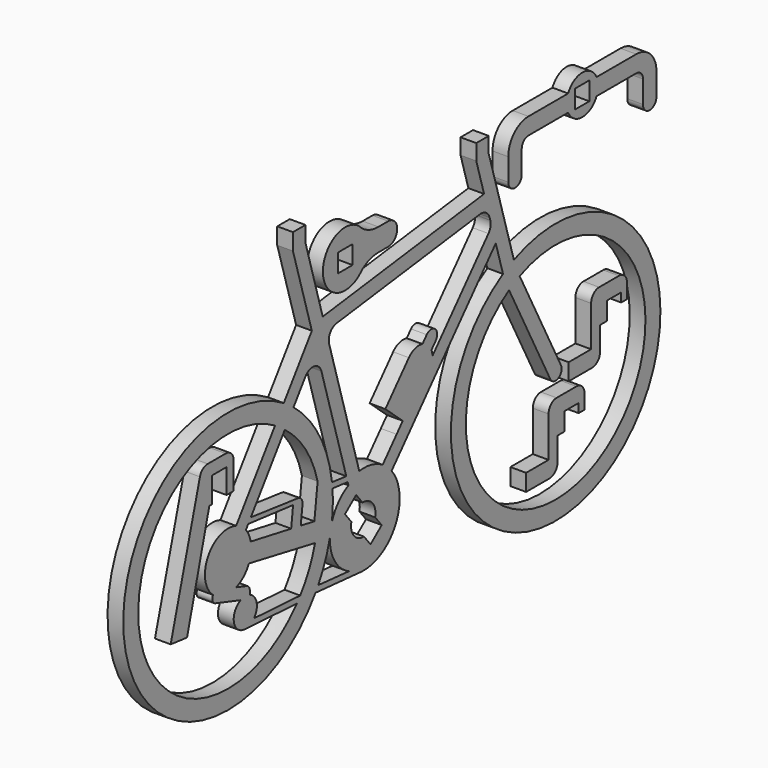
from build123d import *

# Parameters (mm, degrees)
F2_DEPTH = 2.8
F1_W     = 3.286
F1_H     = 3.286
F1_W_2   = 3.2
F1_H_2   = 3.2858568893


# Not quite as in the source:
# - ends of sketch curves that miss each other by under 0.0002 mm in the source are joined
# - a feature names something its author has since deleted; it is built from what else it names


with BuildPart() as f2:
    # F1 (on Right) → F2 (new body)
    with BuildSketch(Plane.YZ):
        with BuildLine():
            Line((-32.7810810621, 40.0630099882), (-28.5785464468, 25.854345194))
            Line((-28.5785464468, 25.854345194), (-34.8295213879, 17.0517607704))
            ThreePointArc((-34.8295213879, 17.0517607704), (-70.0441528649, -7.6634310767), (-27.7561804721, -15.577871613))
            Line((-27.7561804721, -15.577871613), (-17.4309209468, -16.4342678025))
            ThreePointArc((-17.4309209468, -16.4342678025), (-17.421352009, -16.4349690955), (-17.4117713764, -16.4354866475))
            ThreePointArc((-17.4117713764, -16.4354866475), (-9.8783278177, -12.024945839), (-10.8100300989, -3.3452239002))
            Line((-10.8100300989, -3.3452239002), (12.3781786089, 22.9225390659))
            Line((12.3781786089, 22.9225390659), (13.9960358427, 17.4527707038))
            ThreePointArc((13.9960358427, 17.4527707038), (36.2440392418, -23.5369879191), (16.4146126558, 18.6758988393))
            Line((16.4146126558, 18.6758988393), (14.2536723845, 25.9817614853))
            ThreePointArc((14.2536723845, 25.9817614853), (14.2515405676, 25.989045047), (14.2493673209, 25.9963163545))
            Line((14.2493673209, 25.9963163545), (12.7777300944, 30.9717335764))
            Line((12.7777300944, 30.9717335764), (10.8173713638, 37.5995357396))
            Line((10.8173713638, 37.5995357396), (10.8173713638, 40.3995357399))
            Line((10.8173713638, 40.3995357399), (8.037018366, 40.3995357399))
            Line((8.037018366, 40.3995357399), (8.037018366, 37.5995357399))
            Line((8.037018366, 37.5995357399), (9.7773678827, 31.7155655707))
            Line((9.7773678827, 31.7155655707), (-26.1566620581, 27.0789083905))
            Line((-26.1566620581, 27.0789083905), (-30.0007321323, 40.2276701755))
            Line((-30.0007321323, 40.2276701755), (-30.0007321323, 43.0276701755))
            Line((-30.0007321323, 43.0276701755), (-32.7810810175, 43.0276701755))
            Line((-32.7810810175, 43.0276701755), (-32.7810810621, 40.0630099882))
        make_face()
        with BuildLine():
            ThreePointArc((-27.1589419206, -14.6239739066), (-25.6381564049, -11.5709515578), (-24.5785787783, -8.3288797973))
            ThreePointArc((-24.5785787783, -8.3288797973), (-23.4485868958, -12.4014570535), (-20.3032664054, -15.2245273988))
            Line((-20.3032664054, -15.2245273988), (-27.1589419206, -14.6239739066))
        make_face(mode=Mode.SUBTRACT)
        with BuildLine():
            Line((-36.7690909191, 14.3204708989), (-45.438959238, 2.1116157144))
            ThreePointArc((-45.438959238, 2.1116157144), (-51.679021575, -0.1114645339), (-50.5741858599, -6.6429116785))
            ThreePointArc((-50.5741858599, -6.6429116785), (-50.7001368643, -7.5358957288), (-50.0559554, -8.1670172786))
            Line((-50.0559554, -8.1670172786), (-44.4357401431, -9.9504751803))
            ThreePointArc((-44.4357401431, -9.9504751803), (-45.9475994843, -12.7053301629), (-43.682084094, -14.8830318549))
            Line((-43.682084094, -14.8830318549), (-43.4085644782, -14.8992046485))
            Line((-43.4085644782, -14.8992046485), (-31.9213599112, -15.5784253597))
            ThreePointArc((-31.9213599112, -15.5784253597), (-66.9726575865, -5.9191061127), (-36.7690909191, 14.3204708989))
        make_face(mode=Mode.SUBTRACT)
        with BuildLine():
            ThreePointArc((-45.417431414, -7.5410613439), (-43.7533998551, -6.5186996051), (-42.5893207169, -4.9505336974))
            Line((-42.5893207169, -4.9505336974), (-27.8742179451, -7.7233503042))
            ThreePointArc((-27.8742179451, -7.7233503042), (-29.1875288387, -11.3310895929), (-31.1661285889, -14.6213344633))
            Line((-31.1661285889, -14.6213344633), (-41.4453615912, -14.013539249))
            ThreePointArc((-41.4453615912, -14.013539249), (-40.8757428579, -11.7304415251), (-42.3931878811, -9.9320085072))
            Line((-42.3931878811, -9.9320085072), (-42.3931878811, -9.2324187691))
            ThreePointArc((-42.3931878811, -9.2324187691), (-42.5861622295, -8.6419628585), (-43.0905932927, -8.2794348124))
            Line((-43.0905932927, -8.2794348124), (-45.417431414, -7.5410613439))
        make_face(mode=Mode.SUBTRACT)
        with BuildLine():
            Line((-15.5088098858, -12.9576973057), (-16.9709924298, -11.149063212))
            ThreePointArc((-16.9709924298, -11.149063212), (-19.2224479888, -10.1072740955), (-19.7694541503, -7.6875301098))
            Line((-19.7694541503, -7.6875301098), (-21.2014292566, -5.9162608458))
            Line((-21.2014292566, -5.9162608458), (-18.7129342238, -3.9044476159))
            Line((-18.7129342238, -3.9044476159), (-17.2809591175, -5.67571688))
            ThreePointArc((-17.2809591175, -5.67571688), (-15.0295035586, -6.7175059964), (-14.4824973971, -9.1372499821))
            Line((-14.4824973971, -9.1372499821), (-13.0203148531, -10.9458840758))
            Line((-13.0203148531, -10.9458840758), (-15.5088098858, -12.9576973057))
        make_face(mode=Mode.SUBTRACT)
        with BuildLine():
            ThreePointArc((-20.4284332347, -1.7008787129), (-22.713034199, -3.5049348102), (-24.1327228009, -6.0462935497))
            ThreePointArc((-24.1327228009, -6.0462935497), (-23.9042746908, -3.4009611929), (-23.9777551737, -0.7467998497))
            Line((-23.9777551737, -0.7467998497), (-20.6010095051, -1.1174049345))
            Line((-20.6010095051, -1.1174049345), (-20.4284332347, -1.7008787129))
        make_face(mode=Mode.SUBTRACT)
        with BuildLine():
            ThreePointArc((-42.1876674295, -1.6755199445), (-42.5889328041, -0.4877747618), (-43.2651398515, 0.5679224243))
            Line((-43.2651398515, 0.5679224243), (-42.7367221094, 1.3120370351))
            Line((-42.7367221094, 1.3120370351), (-32.7536984043, 0.2163787562))
            Line((-32.7536984043, 0.2163787562), (-33.1812144267, -3.3188663768))
            Line((-33.1812144267, -3.3188663768), (-42.1876674295, -1.6755199445))
        make_face(mode=Mode.SUBTRACT)
        with BuildLine():
            Line((-31.6963693255, 0.8509632025), (-42.1651316758, 2.1169471643))
            Line((-42.1651316758, 2.1169471643), (-34.5952715328, 12.7767776084))
            ThreePointArc((-34.5952715328, 12.7767776084), (-29.9994401309, 7.8666759835), (-27.2914488726, 1.7105775773))
            Line((-27.2914488726, 1.7105775773), (-28.0136806178, -4.2617512446))
            Line((-28.0136806178, -4.2617512446), (-31.0443248868, -3.708770127))
            Line((-31.0443248868, -3.708770127), (-30.6536988323, -0.4785780739))
            ThreePointArc((-30.6536988323, -0.4785780739), (-30.8996770647, 0.402136694), (-31.6963693255, 0.8509632025))
        make_face(mode=Mode.SUBTRACT)
        with BuildLine():
            ThreePointArc((24.5326127574, -3.3329199604), (26.3299626073, -3.9019308276), (26.8989734744, -2.1045809777))
            Line((26.8989734744, -2.1045809777), (17.7069262182, 15.603641135))
            ThreePointArc((17.7069262182, 15.603641135), (34.9283354862, -20.4664558462), (15.3405655012, 14.3753021523))
            Line((15.3405655012, 14.3753021523), (24.5326127574, -3.3329199604))
        make_face(mode=Mode.SUBTRACT)
        with BuildLine():
            ThreePointArc((-29.9983734724, 19.2501011531), (-28.0396469956, 20.0648164886), (-26.4504948685, 18.6594816511))
            Line((-26.4504948685, 18.6594816511), (-20.9085424497, -0.0776477954))
            Line((-20.9085424497, -0.0776477954), (-24.0866021245, 0.2711510752))
            ThreePointArc((-24.0866021245, 0.2711510752), (-26.8907561473, 8.722170153), (-32.6557020014, 15.5080674802))
            Line((-32.6557020014, 15.5080674802), (-29.9983734724, 19.2501011531))
        make_face(mode=Mode.SUBTRACT)
        with BuildLine():
            Line((-18.0250834345, -0.4262562289), (-24.7288519992, 22.2389292241))
            ThreePointArc((-24.7288519992, 22.2389292241), (-24.4867438443, 23.8976541842), (-23.0672336955, 24.7892683327))
            Line((-23.0672336955, 24.7892683327), (8.8532049047, 28.9080418475))
            ThreePointArc((8.8532049047, 28.9080418475), (10.2006691115, 28.6002630517), (11.0266106326, 27.4920175106))
            Line((11.0266106326, 27.4920175106), (11.1717955661, 27.0011658215))
            ThreePointArc((11.1717955661, 27.0011658215), (11.2066686934, 26.0018903312), (10.7533788193, 25.1106575162))
            Line((10.7533788193, 25.1106575162), (-1.7245508843, 10.9755725718))
            ThreePointArc((-1.7245508843, 10.9755725718), (-1.7897327542, 11.4952481661), (-1.9443174541, 11.9956629641))
            Line((-1.9443174541, 11.9956629641), (-0.9945827645, 13.0715289795))
            ThreePointArc((-0.9945827646, 13.0715289795), (-1.1117489129, 14.9531537943), (-2.9933737277, 14.8359876459))
            Line((-2.9933737277, 14.8359876459), (-3.9431084172, 13.7601216304))
            ThreePointArc((-3.9431084172, 13.7601216304), (-5.5866841115, 13.7356227774), (-6.9705428385, 12.8485623057))
            Line((-6.9705428385, 12.8485623057), (-12.2077076552, 6.9158658319))
            Line((-12.2077076552, 6.9158658319), (-8.3300521573, 3.4928151103))
            Line((-8.3300521573, 3.4928151103), (-9.6983886135, 1.9427541226))
            Line((-9.6983886135, 1.9427541226), (-12.8088210603, -1.5807652347))
            ThreePointArc((-12.8088210603, -1.5807652347), (-15.3182270596, -0.5574540272), (-18.0250834345, -0.4262562289))
        make_face(mode=Mode.SUBTRACT)
    extrude(amount=F2_DEPTH)


with BuildPart() as f2b:
    # F1 (on Right) → F2, piece 2 (new body)
    with BuildSketch(Plane.YZ):
        with BuildLine():
            Line((26.1350085661, -17.0272199881), (26.1350085661, -12.8250569627))
            Line((26.1350085661, -12.8250569627), (27.6350085661, -12.8250569627))
            Line((27.6350085661, -12.8250569627), (27.6350085661, -9.6250569627))
            Line((27.6350085661, -9.6250569627), (30.8350085661, -9.6250569627))
            Line((30.8350085661, -9.6250569627), (30.8350085661, -11.2250569627))
            Line((30.8350085661, -11.2250569627), (32.1350085661, -11.2250569627))
            Line((32.1350085661, -11.2250569627), (32.1350085661, -8.6228939372))
            ThreePointArc((32.1350085661, -8.6228939372), (31.6084343077, -7.351631221), (30.3371715916, -6.8250569627))
            Line((30.3371715916, -6.8250569627), (26.1350085661, -6.8250569627))
            Line((26.1350085661, -6.8250569627), (25.9328455406, -6.8250569627))
            ThreePointArc((25.9328455406, -6.8250569627), (24.6615828245, -7.351631221), (24.1350085661, -8.6228939372))
            Line((24.1350085661, -8.6228939372), (24.1350085661, -15.8250569627))
            Line((24.1350085661, -15.8250569627), (19.1350085661, -15.8250569627))
            Line((19.1350085661, -15.8250569627), (19.1350085661, -18.8250569627))
            Line((19.1350085661, -18.8250569627), (24.3371715916, -18.8250569627))
            ThreePointArc((24.3371715916, -18.8250569627), (25.6084343077, -18.2984827043), (26.1350085661, -17.0272199881))
        make_face()
    extrude(amount=F2_DEPTH)


with BuildPart() as f2c:
    # F1 (on Right) → F2, piece 3 (new body)
    with BuildSketch(Plane.YZ):
        with BuildLine():
            Line((-47.7713023129, 14.3973374015), (-51.7613397022, 14.3973374015))
            ThreePointArc((-51.7613397022, 14.3973374015), (-52.8518038089, 14.0305013357), (-53.496568146, 13.077632186))
            Line((-53.496568146, 13.077632186), (-60.0158057756, -10.5528221893))
            Line((-60.0158057756, -10.5528221893), (-56.367214369, -10.9714387513))
            Line((-56.367214369, -10.9714387513), (-51.4058386912, 7.6636058447))
            Line((-51.4058386912, 7.6636058447), (-50.7571436434, 7.6636058447))
            Line((-50.7571436434, 7.6636058447), (-50.7571436434, 12.2000958209))
            Line((-50.7571436434, 12.2000958209), (-47.5571436434, 12.2000958209))
            Line((-47.5571436434, 12.2000958209), (-47.5571436434, 7.799523944))
            Line((-47.5571436434, 7.799523944), (-45.9734653383, 7.799523944))
            Line((-45.9734653383, 7.799523944), (-45.9734653383, 12.599500427))
            ThreePointArc((-45.9734653383, 12.599500427), (-46.5000395967, 13.8707631432), (-47.7713023129, 14.3973374015))
        make_face()
    extrude(amount=F2_DEPTH)


with BuildPart() as f2d:
    # F1 (on Right) → F2, piece 4 (new body)
    with BuildSketch(Plane.YZ):
        with BuildLine():
            ThreePointArc((-11.5660707645, 32.1164598398), (-9.5660707645, 34.1164598398), (-11.5660707645, 36.1164598398))
            Line((-11.5660707645, 36.1164598398), (-13.7510611544, 36.1164598398))
            ThreePointArc((-13.7510611544, 36.1164598398), (-15.6803701734, 36.4351072976), (-17.4047560543, 37.35720427))
            ThreePointArc((-17.4047560543, 37.35720427), (-26.1140103212, 34.1164598398), (-17.4047560543, 30.8757154096))
            ThreePointArc((-17.4047560543, 30.8757154096), (-15.6803701734, 31.7978123821), (-13.7510611544, 32.1164598398))
            Line((-13.7510611544, 32.1164598398), (-11.5660707645, 32.1164598398))
        make_face()
        with Locations((-21.1564369343, 34.1164598398)):
            Rectangle(F1_W, F1_H, mode=Mode.SUBTRACT)
    extrude(amount=F2_DEPTH)


with BuildPart() as f2e:
    # F1 (on Right) → F2, piece 5 (new body)
    with BuildSketch(Plane.YZ):
        with BuildLine():
            ThreePointArc((15.1628487238, 31.3657282359), (16.6628487238, 29.8657282359), (18.1628487238, 31.3657282359))
            Line((18.1628487238, 31.3657282359), (18.1628487238, 35.3657282359))
            ThreePointArc((18.1628487238, 35.3657282359), (18.602188552, 36.4263884077), (19.6628487238, 36.8657282359))
            Line((19.6628487238, 36.8657282359), (28.5005710636, 36.8657282359))
            ThreePointArc((28.5005710636, 36.8657282359), (31.6628487238, 34.8657282359), (34.825126384, 36.8657282359))
            Line((34.825126384, 36.8657282359), (43.6628487238, 36.8657282359))
            ThreePointArc((43.6628487238, 36.8657282359), (44.7235088956, 36.4263884077), (45.1628487238, 35.3657282359))
            Line((45.1628487238, 35.3657282359), (45.1628487238, 31.3657282359))
            ThreePointArc((45.1628487238, 31.3657282359), (46.6628487238, 29.8657282359), (48.1628487238, 31.3657282359))
            Line((48.1628487238, 31.3657282359), (48.1628487238, 35.3657282359))
            ThreePointArc((48.1628487238, 35.3657282359), (46.8448292391, 38.5477087513), (43.6628487238, 39.8657282359))
            Line((43.6628487238, 39.8657282359), (34.825126384, 39.8657282359))
            ThreePointArc((34.825126384, 39.8657282359), (31.6628487238, 41.8657282359), (28.5005710636, 39.8657282359))
            Line((28.5005710636, 39.8657282359), (19.6628487238, 39.8657282359))
            ThreePointArc((19.6628487238, 39.8657282359), (16.4808682084, 38.5477087513), (15.1628487238, 35.3657282359))
            Line((15.1628487238, 35.3657282359), (15.1628487238, 31.3657282359))
        make_face()
        with Locations((31.6199202791, 38.3657282359)):
            Rectangle(F1_W_2, F1_H_2, mode=Mode.SUBTRACT)
    extrude(amount=F2_DEPTH)


with BuildPart() as f2f:
    # F1 (on Right) → F2, piece 6 (new body)
    with BuildSketch(Plane.YZ):
        with BuildLine():
            Line((39.8146519543, 6.6714825634), (35.6124889288, 6.6714825634))
            Line((35.6124889288, 6.6714825634), (35.4103259033, 6.6714825634))
            ThreePointArc((35.4103259033, 6.6714825634), (34.1390631872, 6.144908305), (33.6124889288, 4.8736455889))
            Line((33.6124889288, 4.8736455889), (33.6124889288, -2.3285174366))
            Line((33.6124889288, -2.3285174366), (28.6124889288, -2.3285174366))
            Line((28.6124889288, -2.3285174366), (28.6124889288, -5.3285174366))
            Line((28.6124889288, -5.3285174366), (33.8146519543, -5.3285174366))
            ThreePointArc((33.8146519543, -5.3285174366), (35.0859146704, -4.8019431782), (35.6124889288, -3.5306804621))
            Line((35.6124889288, -3.5306804621), (35.6124889288, 0.6714825634))
            Line((35.6124889288, 0.6714825634), (37.1124889288, 0.6714825634))
            Line((37.1124889288, 0.6714825634), (37.1124889288, 3.8714825634))
            Line((37.1124889288, 3.8714825634), (40.3124889288, 3.8714825634))
            Line((40.3124889288, 3.8714825634), (40.3124889288, 2.2714825634))
            Line((40.3124889288, 2.2714825634), (41.6124889288, 2.2714825634))
            Line((41.6124889288, 2.2714825634), (41.6124889288, 4.8736455889))
            ThreePointArc((41.6124889288, 4.8736455889), (41.0859146704, 6.144908305), (39.8146519543, 6.6714825634))
        make_face()
    extrude(amount=F2_DEPTH)


solid = Compound([f2.part, f2b.part, f2c.part, f2d.part, f2e.part, f2f.part])
